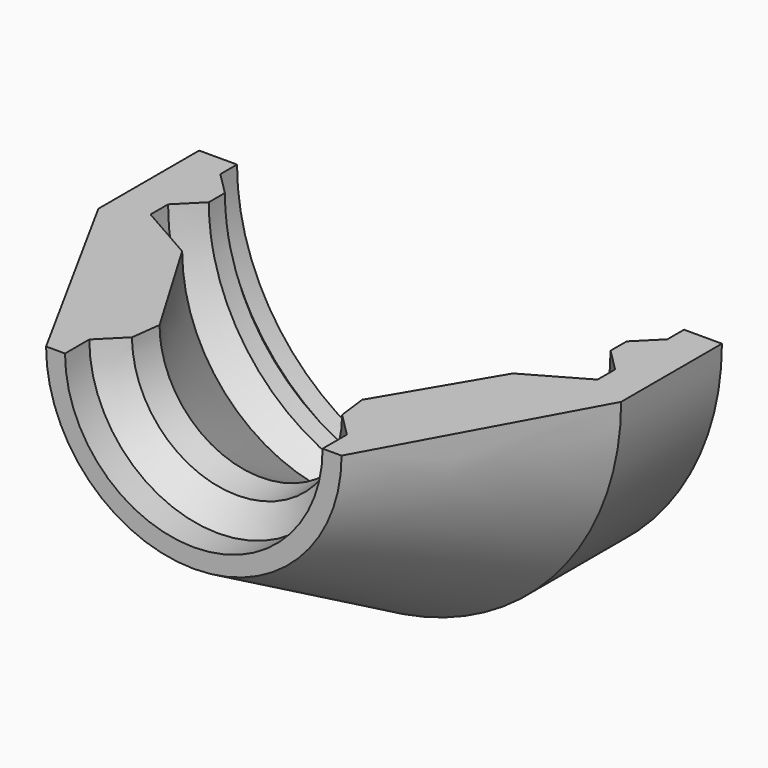
from build123d import *

# Parameters (mm, degrees)
F1_ANGLE     = 180
F2_T4_ANGLE  = 243.2500896942
F2_S5_R      = 11.8
F2_T6_DEPTH  = 16
F3_T4_ANGLE  = 243.6352501502
F3_S5_R      = 11.8
F3_T6_DEPTH  = 16
F4_T4_ANGLE  = 309.1355997924
F4_S5_R      = 6.8
F4_T6_DEPTH  = 11
F4_T10_ANGLE = 243.2500896942
F4_S11_R     = 11.8
F4_T12_DEPTH = 16
F5_SIZE      = 0.75
F6_SIZE      = 1


# Not quite as in the source:
# - a fillet or chamfer that OpenCascade refuses, or shapes differently, is made with other operations: its cross-section is extruded or revolved along the edge and cut away or added
# - a feature names something its author has since deleted; it is built from what else it names


with BuildPart() as f1:
    # F0 (on Top) → F1 (revolve)
    with BuildSketch(Plane.XY):
        Polygon((-11.8, 5.65), (-11.8, 6.65), (-13.8, 6.65), (-13.8, 0), (-7.8, -10.95), (-6.8, -10.95), (-6.8, -9.45), (-4.8, -9.45), (-4.8, -7.45), (-9.8, 1), (-11.8, 1), (-11.8, 2), (-9.8, 2), (-9.8, 5.65), align=None)
    revolve(axis=Axis((0, 0, 0), (0, -1, 0)), revolution_arc=F1_ANGLE)

    # F2: chamfer of 2.1 on 1 edges, made by hand


with BuildPart() as f2_tool2:
    # F2_s3 → F2_t4 (revolve)
    with BuildSketch(Plane(origin=(0, 0, 0), x_dir=(0, 1, 0), z_dir=(0.5243581586, 0, 0.8514978107))):
        Polygon((3.55, 9.8), (5.65, 11.9), (5.65, 9.8), align=None)
    revolve(axis=Axis((0, 5.65, 0), (0, -1, 0)), revolution_arc=F2_T4_ANGLE)

    # F2_s5 → F2_t6 (intersect, symmetric)
    with BuildSketch(Plane.XZ.offset(-4.6)):
        Circle(F2_S5_R)
    extrude(amount=F2_T6_DEPTH, both=True, mode=Mode.INTERSECT)


with BuildPart() as f1_1:
    add(f1.part)

    # F2_t1: cut F2_tool2
    add(f2_tool2.part, mode=Mode.SUBTRACT)

    # F3: chamfer of 2.1 on 1 edges, made by hand


with BuildPart() as f3_tool2:
    # F3_s3 → F3_t4 (revolve)
    with BuildSketch(Plane(origin=(0, 0, 0), x_dir=(0, 1, 0), z_dir=(0.5272172108, 0, 0.849730553))):
        Polygon((-0.8073066866, 8.7305877594), (1, 11.9), (1, 9.8), align=None)
    revolve(axis=Axis((0, 1, 0), (0, -1, 0)), revolution_arc=F3_T4_ANGLE)

    # F3_s5 → F3_t6 (intersect, symmetric)
    with BuildSketch(Plane.XZ.offset(-0.1)):
        Circle(F3_S5_R)
    extrude(amount=F3_T6_DEPTH, both=True, mode=Mode.INTERSECT)


with BuildPart() as f1_2:
    add(f1_1.part)

    # F3_t1: cut F3_tool2
    add(f3_tool2.part, mode=Mode.SUBTRACT)

    # F4: chamfer of 2.1 on 2 edges, made by hand


with BuildPart() as f4_tool2:
    # F4_s3 → F4_t4 (revolve)
    with BuildSketch(Plane(origin=(0, 0, 0), x_dir=(0, 1, 0), z_dir=(0.9030940896, 0, 0.4294427381))):
        Polygon((-7.35, 4.8), (-9.45, 6.9), (-9.45, 4.8), align=None)
    revolve(axis=Axis((0, -9.45, 0), (0, -1, 0)), revolution_arc=F4_T4_ANGLE)

    # F4_s5 → F4_t6 (intersect, symmetric)
    with BuildSketch(Plane.XZ.offset(8.4)):
        Circle(F4_S5_R)
    extrude(amount=F4_T6_DEPTH, both=True, mode=Mode.INTERSECT)


with BuildPart() as f1_3:
    add(f1_2.part)

    # F4_t1: cut F4_tool2
    add(f4_tool2.part, mode=Mode.SUBTRACT)


with BuildPart() as f4_tool8:
    # F4_s9 → F4_t10 (revolve)
    with BuildSketch(Plane(origin=(0, 0, 0), x_dir=(0, 1, 0), z_dir=(0.5243581586, 0, 0.8514978107))):
        Polygon((4.1, 9.8), (2, 11.9), (2, 9.8), align=None)
    revolve(axis=Axis((0, 2, 0), (0, -1, 0)), revolution_arc=F4_T10_ANGLE)

    # F4_s11 → F4_t12 (intersect, symmetric)
    with BuildSketch(Plane.XZ.offset(-3)):
        Circle(F4_S11_R)
    extrude(amount=F4_T12_DEPTH, both=True, mode=Mode.INTERSECT)


with BuildPart() as f1_4:
    add(f1_3.part)

    # F4_t7: cut F4_tool8
    add(f4_tool8.part, mode=Mode.SUBTRACT)

    # F5
    f5_edges = [f1_4.edges().sort_by_distance(p)[0] for p in [
        (0, 3.825, -10.075),
    ]]
    chamfer(f5_edges, length=F5_SIZE)

    # F6
    f6_edges = [f1_4.edges().sort_by_distance(p)[0] for p in [
        (0, -7.387175, -4.837175),
    ]]
    chamfer(f6_edges, length=F6_SIZE)


solid = f1_4.part
